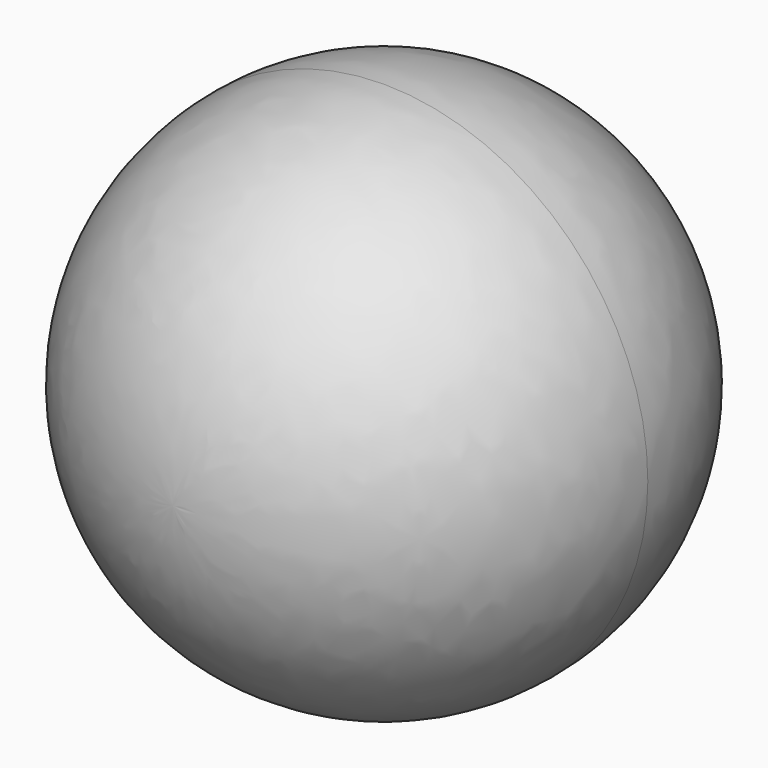
from build123d import *

# Parameters (mm, degrees)
F0_R          = 50
F1_DEPTH      = 50
F1_DEPTH_BACK = 50
F2_R          = 49.99999
F3_T          = 5


# Not quite as in the source:
# - a fillet or chamfer is up to 0.001 mm smaller than in the source, because OpenCascade refuses the exact size


with BuildPart() as f1:
    # F0 (on Front) → F1 (new body, two sides)
    with BuildSketch(Plane.XZ) as f1_sk:
        Circle(F0_R)
    extrude(amount=F1_DEPTH)
    extrude(f1_sk.sketch, amount=-F1_DEPTH_BACK)

    # F2 (radius 50 in the source; OpenCascade refuses exactly that, so slightly less here)
    f2_edges = [f1.edges().sort_by_distance(p)[0] for p in [
        (-50, 50, 0),
        (-50, -50, 0),
    ]]
    fillet(f2_edges, radius=F2_R)

    # F3 (hollow, outwards: the wall grows on the outside; the body as it was is the cavity)
    f3_inside = f1.part
    offset(amount=F3_T)
    add(f3_inside, mode=Mode.SUBTRACT)


solid = f1.part
